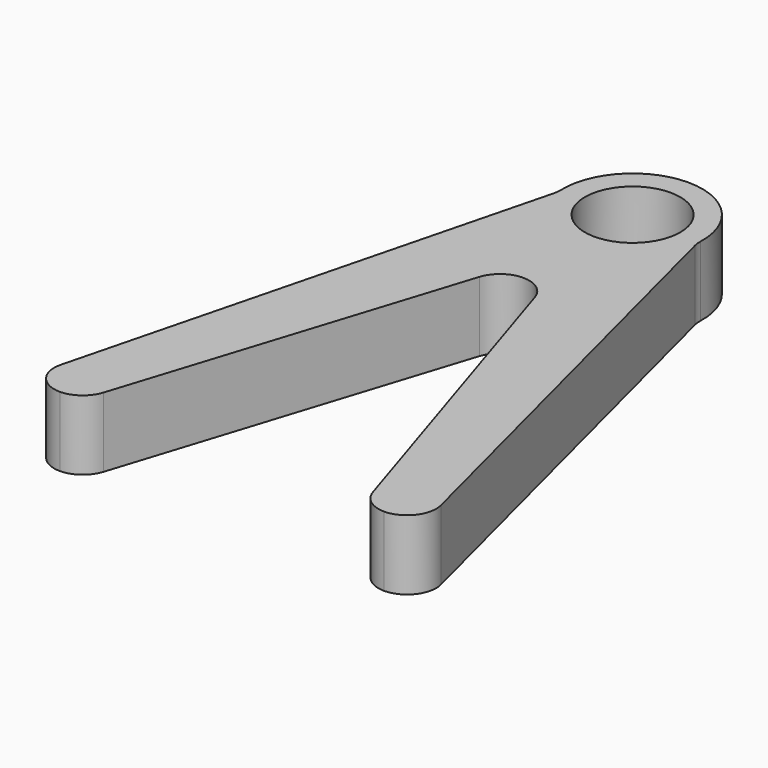
from build123d import *

# Parameters (mm, degrees)
F0_R        = 8.2
F1_DEPTH    = 12
F2_DEPTH    = 2
F3_T1_DEPTH = 12
F3_T3_DEPTH = 30.2772195225
F3_T5_DEPTH = 44.2039362688


# Not quite as in the source:
# - a fillet or chamfer that OpenCascade refuses, or shapes differently, is made with other operations: its cross-section is extruded or revolved along the edge and cut away or added


with BuildPart() as f1:
    # F0 (on Top) → F1 (new body)
    with BuildSketch(Plane.XY):
        with BuildLine():
            Line((34.2691161265, 0), (11.9548385252, 87.1898676173))
            ThreePointArc((11.9548385252, 87.1898676173), (0, 100.2299809946), (-11.9548385252, 87.1898676173))
            Line((-11.9548385252, 87.1898676173), (-34.2691161265, 0))
            Line((-34.2691161265, 0), (-24.2691161265, 0))
            Line((-24.2691161265, 0), (0, 76.2299809946))
            Line((0, 76.2299809946), (24.2691161265, 0))
            Line((24.2691161265, 0), (34.2691161265, 0))
        make_face()
        with Locations((0, 88.2299809946)):
            Circle(F0_R, mode=Mode.SUBTRACT)
    extrude(amount=F1_DEPTH)

    # F0 (on Top) → F2 (join)
    with BuildSketch(Plane.XY):
        with Locations((0, 88.2299809946)):
            Circle(F0_R)
    extrude(amount=F2_DEPTH)

    # F3: fillet of radius 5 on 7 edges, made by hand

    # F3_s2 → F3_t1 (join)
    with BuildSketch(Plane.XY):
        with BuildLine():
            ThreePointArc((-4.7643738122, 61.2649479353), (0, 64.7481281774), (4.7643738122, 61.2649479353))
            Line((4.7643738122, 61.2649479353), (0, 76.2299809946))
            Line((0, 76.2299809946), (-4.7643738122, 61.2649479353))
        make_face()
        with BuildLine():
            ThreePointArc((11.9936747891, 87.8404106503), (12.0207340622, 87.1339702047), (12.1471577503, 86.4384075845))
            Line((12.1471577503, 86.4384075845), (11.9548385252, 87.1898676173))
            ThreePointArc((11.9548385252, 87.1898676173), (11.9786737183, 87.5148754431), (11.9936747891, 87.8404106503))
        make_face()
        with BuildLine():
            ThreePointArc((-12.1471577503, 86.4384075845), (-12.0207340622, 87.1339702047), (-11.9936747891, 87.8404106503))
            ThreePointArc((-11.9936747891, 87.8404106503), (-11.9786737183, 87.5148754431), (-11.9548385252, 87.1898676173))
            Line((-11.9548385252, 87.1898676173), (-12.1471577503, 86.4384075845))
        make_face()
    extrude(amount=F3_T1_DEPTH)

    # F3_s4 → F3_t3 (cut)
    with BuildSketch(Plane.XY.offset(-9.1386097613)):
        with BuildLine():
            ThreePointArc((-27.924560031, 0), (-24.9736363442, 0.96365891), (-23.1601862189, 3.4831802421))
            Line((-23.1601862189, 3.4831802421), (-24.2691161265, 0))
            Line((-24.2691161265, 0), (-27.924560031, 0))
        make_face()
        with BuildLine():
            ThreePointArc((23.1601862189, 3.4831802421), (24.9736363442, 0.96365891), (27.924560031, 0))
            Line((27.924560031, 0), (24.2691161265, 0))
            Line((24.2691161265, 0), (23.1601862189, 3.4831802421))
        make_face()
    extrude(amount=F3_T3_DEPTH, mode=Mode.SUBTRACT)

    # F3_s6 → F3_t5 (cut)
    with BuildSketch(Plane.XY.offset(-16.1019681344)):
        with BuildLine():
            ThreePointArc((-27.8283288728, 0), (-31.7779117903, 1.9339284455), (-32.6722104071, 6.239682089))
            Line((-32.6722104071, 6.239682089), (-34.2691161265, 0))
            Line((-34.2691161265, 0), (-27.8283288728, 0))
        make_face()
        with BuildLine():
            ThreePointArc((27.8283288728, 0), (31.7779117903, 1.9339284455), (32.6722104071, 6.239682089))
            Line((32.6722104071, 6.239682089), (34.2691161265, 0))
            Line((34.2691161265, 0), (27.8283288728, 0))
        make_face()
    extrude(amount=F3_T5_DEPTH, mode=Mode.SUBTRACT)


solid = f1.part
